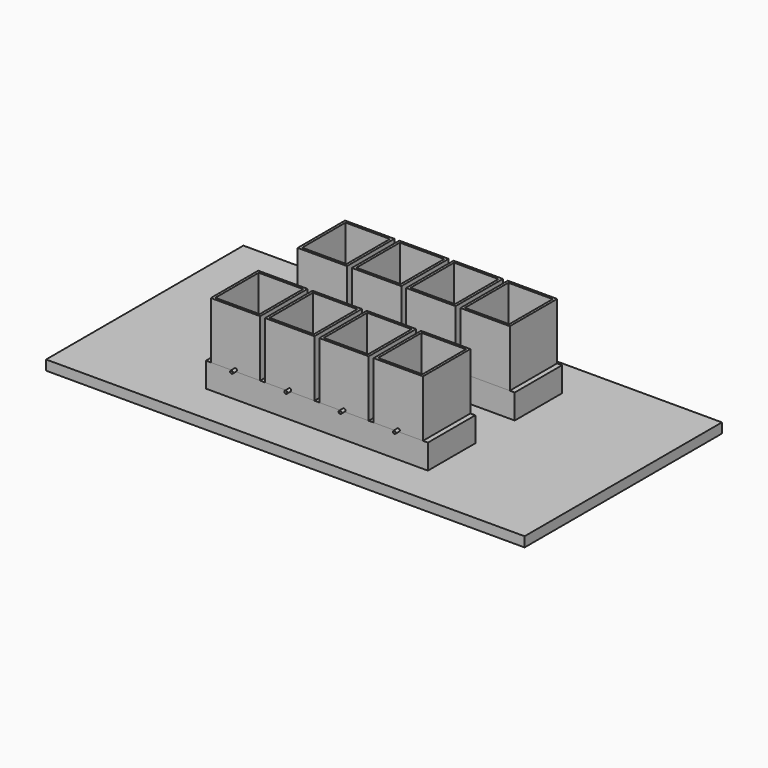
from build123d import *

# Parameters (mm, degrees)
F0_W     = 9700
F0_H     = 5000
F1_DEPTH = 200
F2_W     = 4500
F2_H     = 1200
F3_DEPTH = 500
F4_W     = 1000
F4_H     = 1200
F4_W_2   = 900
F4_H_2   = 1100
F5_DEPTH = 1150
F6_R     = 30
F6_R_2   = 25.4
F7_DEPTH = 100
F8_R     = 30
F8_R_2   = 25.4
F9_DEPTH = 100


with BuildPart() as f1:
    # F0 (on Top) → F1 (new body)
    with BuildSketch(Plane.XY):
        with Locations((4850, 2500)):
            Rectangle(F0_W, F0_H)
    extrude(amount=F1_DEPTH)

    # F2 (on face) → F3 (join)
    with BuildSketch(Plane.XY.offset(200)):
        with Locations((4850, 1400)):
            Rectangle(F2_W, F2_H)
        with Locations((4850, 3600)):
            Rectangle(F2_W, F2_H)
    extrude(amount=F3_DEPTH)


with BuildPart() as f5:
    # F4 (on face) → F5 (new body)
    with BuildSketch(Plane.XY.offset(700)):
        with Locations((3200, 3600)):
            Rectangle(F4_W, F4_H)
        with Locations((3200, 3600)):
            Rectangle(F4_W_2, F4_H_2, mode=Mode.SUBTRACT)
    extrude(amount=F5_DEPTH)

    # F8 (on face) → F9, piece 4 (join)
    with BuildSketch(Plane(origin=(0, 4200, 0), x_dir=(-1, 0, 0), z_dir=(0, 1, 0))):
        with Locations((-3200, 730)):
            Circle(F8_R)
        with Locations((-3200, 730)):
            Circle(F8_R_2, mode=Mode.SUBTRACT)
    extrude(amount=F9_DEPTH)


with BuildPart() as f5b:
    # F4 (on face) → F5, piece 2 (new body)
    with BuildSketch(Plane.XY.offset(700)):
        with Locations((4300, 3600)):
            Rectangle(F4_W, F4_H)
        with Locations((4300, 3600)):
            Rectangle(F4_W_2, F4_H_2, mode=Mode.SUBTRACT)
    extrude(amount=F5_DEPTH)

    # F8 (on face) → F9, piece 3 (join)
    with BuildSketch(Plane(origin=(0, 4200, 0), x_dir=(-1, 0, 0), z_dir=(0, 1, 0))):
        with Locations((-4300, 730)):
            Circle(F8_R)
        with Locations((-4300, 730)):
            Circle(F8_R_2, mode=Mode.SUBTRACT)
    extrude(amount=F9_DEPTH)


with BuildPart() as f5c:
    # F4 (on face) → F5, piece 3 (new body)
    with BuildSketch(Plane.XY.offset(700)):
        with Locations((5400, 3600)):
            Rectangle(F4_W, F4_H)
        with Locations((5400, 3600)):
            Rectangle(F4_W_2, F4_H_2, mode=Mode.SUBTRACT)
    extrude(amount=F5_DEPTH)

    # F8 (on face) → F9, piece 2 (join)
    with BuildSketch(Plane(origin=(0, 4200, 0), x_dir=(-1, 0, 0), z_dir=(0, 1, 0))):
        with Locations((-5400, 730)):
            Circle(F8_R)
        with Locations((-5400, 730)):
            Circle(F8_R_2, mode=Mode.SUBTRACT)
    extrude(amount=F9_DEPTH)


with BuildPart() as f5d:
    # F4 (on face) → F5, piece 4 (new body)
    with BuildSketch(Plane.XY.offset(700)):
        with Locations((6500, 3600)):
            Rectangle(F4_W, F4_H)
        with Locations((6500, 3600)):
            Rectangle(F4_W_2, F4_H_2, mode=Mode.SUBTRACT)
    extrude(amount=F5_DEPTH)

    # F8 (on face) → F9 (join)
    with BuildSketch(Plane(origin=(0, 4200, 0), x_dir=(-1, 0, 0), z_dir=(0, 1, 0))):
        with Locations((-6500, 730)):
            Circle(F8_R)
        with Locations((-6500, 730)):
            Circle(F8_R_2, mode=Mode.SUBTRACT)
    extrude(amount=F9_DEPTH)


with BuildPart() as f5e:
    # F4 (on face) → F5, piece 5 (new body)
    with BuildSketch(Plane.XY.offset(700)):
        with Locations((4300, 1400)):
            Rectangle(F4_W, F4_H)
        with Locations((4300, 1400)):
            Rectangle(F4_W_2, F4_H_2, mode=Mode.SUBTRACT)
    extrude(amount=F5_DEPTH)

    # F6 (on face) → F7, piece 2 (join)
    with BuildSketch(Plane.XZ.offset(-800)):
        with Locations((4300, 730)):
            Circle(F6_R)
        with Locations((4300, 730)):
            Circle(F6_R_2, mode=Mode.SUBTRACT)
    extrude(amount=F7_DEPTH)


with BuildPart() as f5f:
    # F4 (on face) → F5, piece 6 (new body)
    with BuildSketch(Plane.XY.offset(700)):
        with Locations((6500, 1400)):
            Rectangle(F4_W, F4_H)
        with Locations((6500, 1400)):
            Rectangle(F4_W_2, F4_H_2, mode=Mode.SUBTRACT)
    extrude(amount=F5_DEPTH)

    # F6 (on face) → F7, piece 4 (join)
    with BuildSketch(Plane.XZ.offset(-800)):
        with Locations((6500, 730)):
            Circle(F6_R)
        with Locations((6500, 730)):
            Circle(F6_R_2, mode=Mode.SUBTRACT)
    extrude(amount=F7_DEPTH)


with BuildPart() as f5g:
    # F4 (on face) → F5, piece 7 (new body)
    with BuildSketch(Plane.XY.offset(700)):
        with Locations((3200, 1400)):
            Rectangle(F4_W, F4_H)
        with Locations((3200, 1400)):
            Rectangle(F4_W_2, F4_H_2, mode=Mode.SUBTRACT)
    extrude(amount=F5_DEPTH)

    # F6 (on face) → F7 (join)
    with BuildSketch(Plane.XZ.offset(-800)):
        with Locations((3200, 730)):
            Circle(F6_R)
        with Locations((3200, 730)):
            Circle(F6_R_2, mode=Mode.SUBTRACT)
    extrude(amount=F7_DEPTH)


with BuildPart() as f5h:
    # F4 (on face) → F5, piece 8 (new body)
    with BuildSketch(Plane.XY.offset(700)):
        with Locations((5400, 1400)):
            Rectangle(F4_W, F4_H)
        with Locations((5400, 1400)):
            Rectangle(F4_W_2, F4_H_2, mode=Mode.SUBTRACT)
    extrude(amount=F5_DEPTH)

    # F6 (on face) → F7, piece 3 (join)
    with BuildSketch(Plane.XZ.offset(-800)):
        with Locations((5400, 730)):
            Circle(F6_R)
        with Locations((5400, 730)):
            Circle(F6_R_2, mode=Mode.SUBTRACT)
    extrude(amount=F7_DEPTH)


solid = Compound([f1.part, f5.part, f5b.part, f5c.part, f5d.part, f5e.part, f5f.part, f5g.part, f5h.part])
